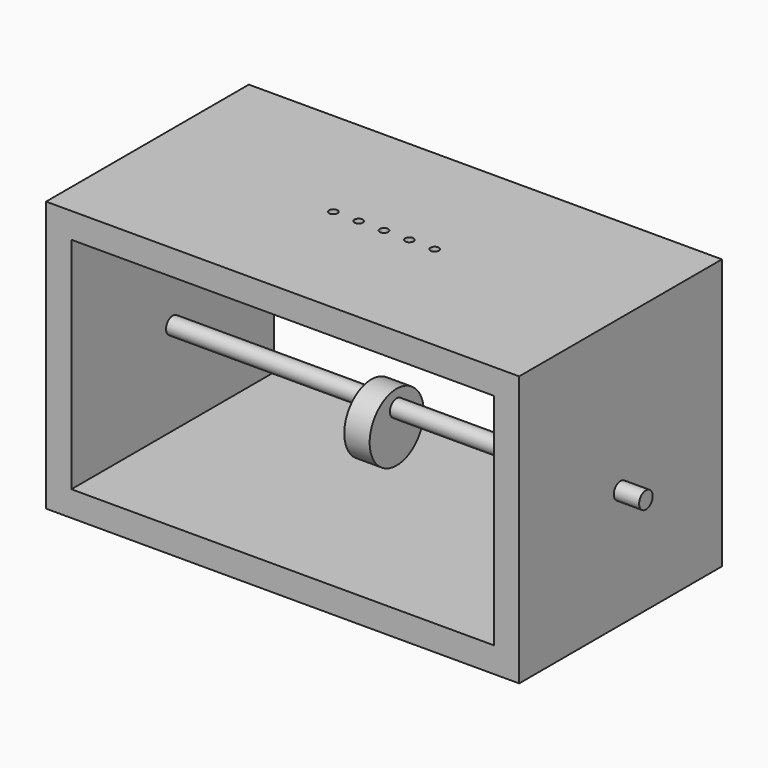
from build123d import *

# Parameters (mm, degrees)
F0_W      = 355.6
F0_H      = 203.2
F0_W_2    = 317.5
F0_H_2    = 165.1
F1_DEPTH  = 95.25
F2_R      = 6.35
F3_DEPTH  = 355.601
F4_R      = 50.8
F4_R_2    = 6.35
F5_DEPTH  = 19.05
F6_R      = 6.35
F7_DEPTH  = 19.05
F9_R      = 6.35
F10_DEPTH = 355.6
F11_R     = 25.4
F11_R_2   = 6.35
F12_DEPTH = 9.525
F13_R     = 3.175
F14_DEPTH = 19.05


# Not quite as in the source:
# - the program builds the solid bodies; features that only make, move or delete a surface that nothing else refers to are left out


with BuildPart() as f1:
    # F0 (on Front) → F1 (new body, symmetric)
    with BuildSketch(Plane.XZ):
        Rectangle(F0_W, F0_H)
        Rectangle(F0_W_2, F0_H_2, mode=Mode.SUBTRACT)
    extrude(amount=F1_DEPTH, both=True)

    # F2 (on face) → F3 (cut, through all)
    with BuildSketch(Plane(origin=(-177.8, 0, 0), x_dir=(0, -1, 0), z_dir=(-1, 0, 0))):
        with Locations((0, -12.7)):
            Circle(F2_R)
    extrude(amount=-F3_DEPTH, mode=Mode.SUBTRACT)

    # F13 (on face) → F14 (cut, through all)
    with BuildSketch(Plane.XY.offset(101.6)):
        with Locations((-38.1, 0)):
            Circle(F13_R)
        with Locations((-19.05, 0)):
            Circle(F13_R)
        Circle(F13_R)
        with Locations((19.05, 0)):
            Circle(F13_R)
        with Locations((38.1, 0)):
            Circle(F13_R)
    extrude(amount=-F14_DEPTH, mode=Mode.SUBTRACT)


with BuildPart() as f5:
    # F4 (on face) → F5 (new body)
    with BuildSketch(Plane(origin=(-177.8, 0, 0), x_dir=(0, -1, 0), z_dir=(-1, 0, 0))):
        with Locations((0, -12.7)):
            Circle(F4_R)
        with Locations((0, -12.7)):
            Circle(F4_R_2, mode=Mode.SUBTRACT)
    extrude(amount=F5_DEPTH)

    # F6 (on face) → F7 (cut, through all)
    with BuildSketch(Plane(origin=(-196.85, 0, 0), x_dir=(0, -1, 0), z_dir=(-1, 0, 0))):
        with Locations((0, 25.4)):
            Circle(F6_R)
    extrude(amount=-F7_DEPTH, mode=Mode.SUBTRACT)


with BuildPart() as f10:
    # F9 (on face) → F10 (new body)
    with BuildSketch(Plane.YZ.offset(-158.75)):
        with Locations((0, -12.7)):
            Circle(F9_R)
    extrude(amount=F10_DEPTH)


with BuildPart() as f12:
    # F11 (on Right) → F12 (new body, symmetric)
    with BuildSketch(Plane.YZ):
        with Locations((0, -25.4)):
            Circle(F11_R)
        with Locations((0, -12.7)):
            Circle(F11_R_2, mode=Mode.SUBTRACT)
    extrude(amount=F12_DEPTH, both=True)


solid = Compound([f1.part, f5.part, f10.part, f12.part])
